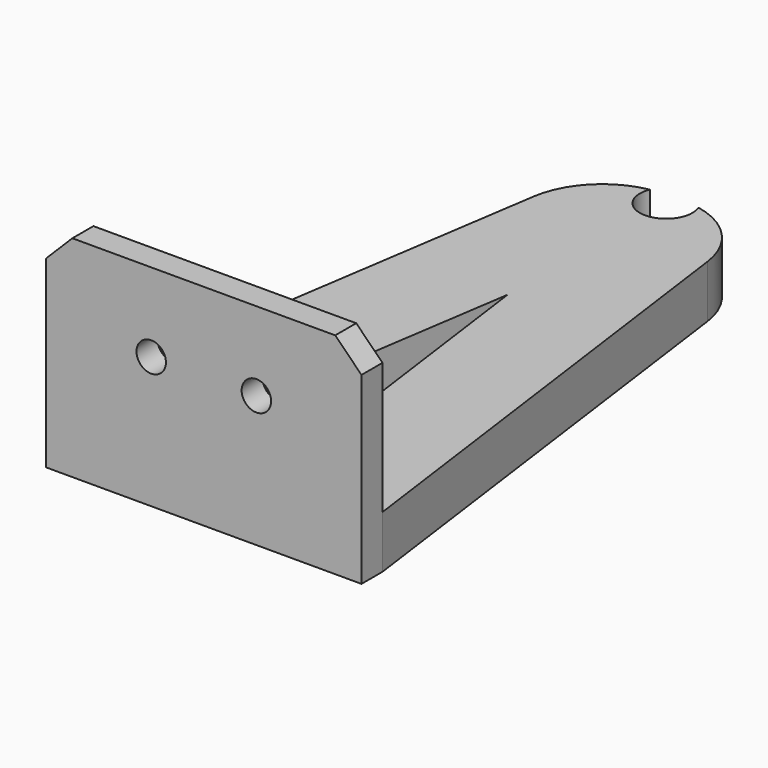
from build123d import *

# Parameters (mm, degrees)
F1_DEPTH    = 10
F2_DEPTH    = 40
F3_R        = 2.8
F4_DEPTH    = 5
F5_T1_DEPTH = 80.8666856224
F5_T3_DEPTH = 81.0791317508
F6_SIZE     = 5


# Not quite as in the source:
# - a fillet or chamfer that OpenCascade refuses, or shapes differently, is made with other operations: its cross-section is extruded or revolved along the edge and cut away or added


with BuildPart() as f1:
    # F0 (on Top) → F1 (new body)
    with BuildSketch(Plane.XY):
        with BuildLine():
            Line((-43.5517183587, 35.5855710396), (-59.7826302073, -71.725967915))
            Line((-59.7826302073, -71.725967915), (-38.9637436029, -71.725967915))
            Line((-38.9637436029, -71.725967915), (-28.9527400952, -5.5376845384))
            Line((-28.9527400952, -5.5376845384), (-19.966132513, -71.725967915))
            Line((-19.966132513, -71.725967915), (0.2173697927, -71.725967915))
            Line((0.2173697927, -71.725967915), (-14.3378386668, 35.4762497537))
            Line((-14.3378386668, 35.4762497537), (-24.3294449803, 34.076745098))
            ThreePointArc((-24.3294449803, 34.076745098), (-28.9527400952, 27.172764457), (-33.57603521, 34.076745098))
            Line((-33.57603521, 34.076745098), (-43.5517183587, 35.5855710396))
        make_face()
    extrude(amount=F1_DEPTH)

    # F0 (on Top) → F2 (join)
    with BuildSketch(Plane.XY):
        Polygon((-38.9637436029, -71.725967915), (-59.7826302073, -71.725967915), (-59.7826302073, -76.725967915), (0.2173697927, -76.725967915), (0.2173697927, -71.725967915), (-19.966132513, -71.725967915), align=None)
    extrude(amount=F2_DEPTH)

    # F3 (on face) → F4 (cut, through all)
    with BuildSketch(Plane(origin=(0, -71.725967915, 0), x_dir=(-1, 0, 0), z_dir=(0, 1, 0))):
        with Locations((39.7826302073, 25)):
            Circle(F3_R)
        with Locations((19.7826302073, 25)):
            Circle(F3_R)
    extrude(amount=-F4_DEPTH, mode=Mode.SUBTRACT)

    # F5: fillet of radius 15 on 2 edges, made by hand

    # F5_s2 → F5_t1 (cut)
    with BuildSketch(Plane.XY.offset(-35.4333428112)):
        with BuildLine():
            ThreePointArc((-33.57603521, 34.076745098), (-41.6218227772, 29.7568391026), (-45.6713333114, 21.5716237836))
            Line((-45.6713333114, 21.5716237836), (-43.5517183587, 35.5855710396))
            Line((-43.5517183587, 35.5855710396), (-33.57603521, 34.076745098))
        make_face()
    extrude(amount=F5_T1_DEPTH, mode=Mode.SUBTRACT)

    # F5_s4 → F5_t3 (cut)
    with BuildSketch(Plane.XY.offset(-35.5395658754)):
        with BuildLine():
            ThreePointArc((-12.4252559054, 21.3896694023), (-16.3501492828, 29.6353150708), (-24.3294449803, 34.076745098))
            Line((-24.3294449803, 34.076745098), (-14.3378386668, 35.4762497537))
            Line((-14.3378386668, 35.4762497537), (-12.4252559054, 21.3896694023))
        make_face()
    extrude(amount=F5_T3_DEPTH, mode=Mode.SUBTRACT)

    # F6
    f6_edges = [f1.edges().sort_by_distance(p)[0] for p in [
        (0.21737, -74.225968, 40),
        (-59.78263, -74.225968, 40),
    ]]
    chamfer(f6_edges, length=F6_SIZE)


solid = f1.part
